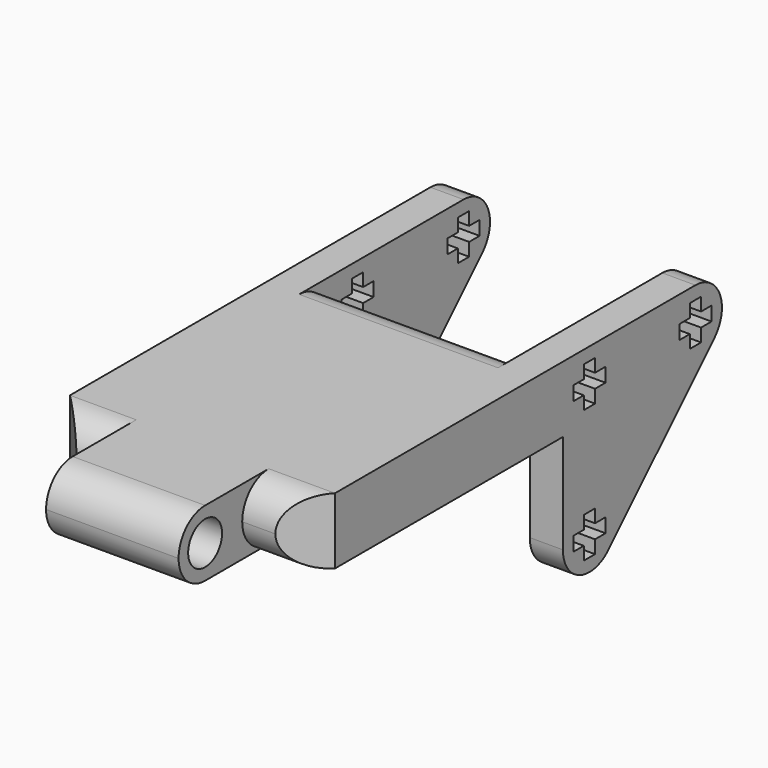
from build123d import *

# Parameters (mm, degrees)
F1_DEPTH = 7.9375
F2_R     = 3.96874
F3_W     = 3.96875
F3_H     = 23.8125
F4_DEPTH = 15.875
F5_W     = 1.56845
F5_H     = 1.6891
F5_W_2   = 1.6891
F5_H_2   = 1.56845
F5_R     = 2.54
F6_DEPTH = 31.75
F8_DEPTH = 7.9375


# Not quite as in the source:
# - a fillet or chamfer is up to 0.001 mm smaller than in the source, because OpenCascade refuses the exact size


with BuildPart() as f1:
    # F0 (on Top) → F1 (new body)
    with BuildSketch(Plane.XY):
        Polygon((0, 0), (0, -9.525), (15.875, -9.525), (15.875, 0), (23.8125, 0), (23.8125, 61.9125), (19.84375, 61.9125), (19.84375, 37.30625), (-3.96875, 37.30625), (-3.96875, 61.9125), (-7.9375, 61.9125), (-7.9375, 0), align=None)
    extrude(amount=F1_DEPTH)

    # F2 (radius 3.96875 in the source; OpenCascade refuses exactly that, so slightly less here)
    f2_edges = [f1.edges().sort_by_distance(p)[0] for p in [
        (19.84375, 0, 7.9375),
        (19.84375, 0, 0),
        (7.9375, -9.525, 0),
        (7.9375, -9.525, 7.9375),
        (-3.96875, 0, 7.9375),
        (-3.96875, 0, 0),
        (-5.953125, 61.9125, 7.9375),
        (7.9375, 37.30625, 0),
        (7.9375, 37.30625, 7.9375),
        (21.828125, 61.9125, 7.9375),
    ]]
    fillet(f2_edges, radius=F2_R)

    # F3 (on face) → F4 (join)
    with BuildSketch(Plane(origin=(0, 0, 0), x_dir=(1, 0, 0), z_dir=(0, 0, -1))):
        with Locations((21.828125, -50.00625)):
            Rectangle(F3_W, F3_H)
        with Locations((-5.953125, -50.00625)):
            Rectangle(F3_W, F3_H)
    extrude(amount=F4_DEPTH)

    # F5 (on face) → F6 (cut, through all)
    with BuildSketch(Plane.YZ.offset(23.8125)):
        with BuildLine():
            Line((38.1, -15.875), (42.06875, -15.875))
            ThreePointArc((42.06875, -15.875), (39.2624199622, -14.7125800378), (38.1, -11.90625))
            Line((38.1, -11.90625), (38.1, -15.875))
        make_face()
        with BuildLine():
            Line((42.06875, -15.875), (61.9125, -15.875))
            Line((61.9125, -15.875), (61.9125, 3.96875))
            ThreePointArc((61.9125, 3.96875), (61.6103968947, 2.4499751278), (60.7500800378, 1.1624199622))
            Line((60.7500800378, 1.1624199622), (44.8750800378, -14.7125800378))
            ThreePointArc((44.8750800378, -14.7125800378), (43.5875248722, -15.5728968947), (42.06875, -15.875))
        make_face()
        with Locations((43.697525, -11.90625)):
            Rectangle(F5_W, F5_H)
        with Locations((42.06875, -11.90625)):
            Rectangle(F5_W_2, F5_H)
        with Locations((42.06875, -10.277475)):
            Rectangle(F5_W_2, F5_H_2)
        with Locations((40.439975, -11.90625)):
            Rectangle(F5_W, F5_H)
        with Locations((42.06875, -13.535025)):
            Rectangle(F5_W_2, F5_H_2)
        with Locations((57.94375, 5.597525)):
            Rectangle(F5_W_2, F5_H_2)
        with Locations((57.94375, 3.96875)):
            Rectangle(F5_W_2, F5_H)
        with Locations((56.314975, 3.96875)):
            Rectangle(F5_W, F5_H)
        with Locations((59.572525, 3.96875)):
            Rectangle(F5_W, F5_H)
        with Locations((57.94375, 2.339975)):
            Rectangle(F5_W_2, F5_H_2)
        with Locations((42.06875, 2.339975)):
            Rectangle(F5_W_2, F5_H_2)
        with Locations((42.06875, 3.96875)):
            Rectangle(F5_W_2, F5_H)
        with Locations((43.697525, 3.96875)):
            Rectangle(F5_W, F5_H)
        with Locations((40.439975, 3.96875)):
            Rectangle(F5_W, F5_H)
        with Locations((42.06875, 5.597525)):
            Rectangle(F5_W_2, F5_H_2)
        with Locations((-5.55625, 3.96875)):
            Circle(F5_R)
    extrude(amount=-F6_DEPTH, mode=Mode.SUBTRACT)

    # F7 (on face) → F8 (cut, through all)
    with BuildSketch(Plane.XY.offset(7.9375)):
        Polygon((19.84375, 0), (23.8125, 0), (23.8125, 3.96875), align=None)
        Polygon((-7.9375, 3.96875), (-7.9375, 0), (-3.96875, 0), align=None)
    extrude(amount=-F8_DEPTH, mode=Mode.SUBTRACT)


solid = f1.part
